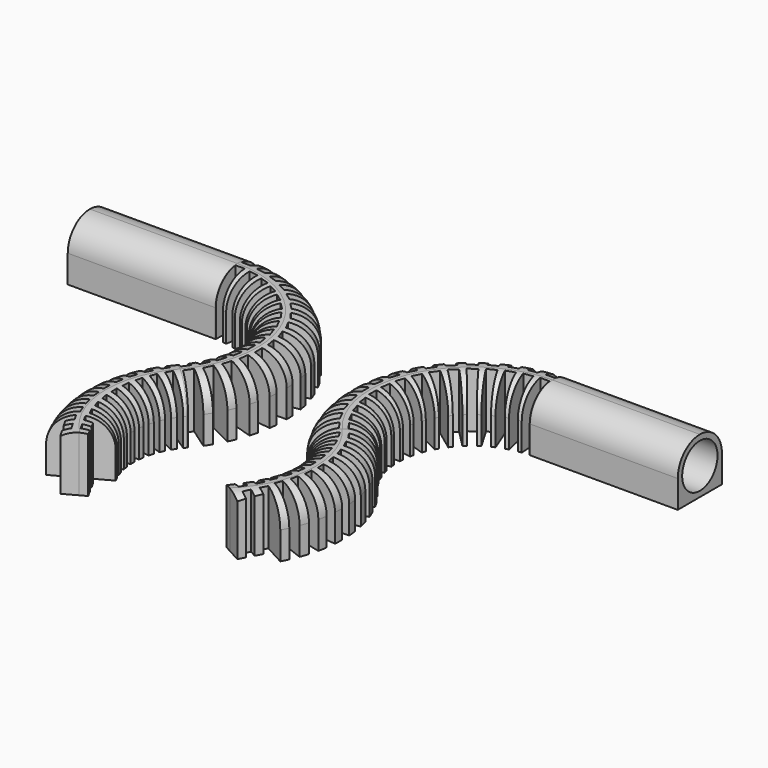
from build123d import *

# Parameters (mm, degrees)
F1_DEPTH = 15
F2_R     = 7.49999
F4_DEPTH = 15.0010001
F6_DEPTH = 25
F8_R     = 6
F9_DEPTH = 18


# Not quite as in the source:
# - a fillet or chamfer is up to 0.001 mm smaller than in the source, because OpenCascade refuses the exact size


with BuildPart() as f1:
    # F0 (on Top) → F1 (new body)
    with BuildSketch(Plane.XY):
        with BuildLine():
            Line((-77.8706056387, 57.7877178192), (-77.8706056387, 42.7877178192))
            Line((-77.8706056387, 42.7877178192), (-37.8706056387, 42.7877178192))
            ThreePointArc((-37.8706056387, 42.7877178192), (-19.7095136662, 31.1417172644), (-22.7163445519, 9.7778796274))
            ThreePointArc((-22.7163445519, 9.7778796274), (-30.7004171335, -8.6672744837), (-26.8147589411, -28.3870814195))
            Line((-26.8147589411, -28.3870814195), (-21.1033173398, -25.2839110882))
            Line((-21.1033173398, -25.2839110882), (-20.1484983127, -27.041272925))
            Line((-20.1484983127, -27.041272925), (-21.9058601495, -27.9960919522))
            Line((-21.9058601495, -27.9960919522), (-20.9510411223, -29.7534537889))
            Line((-20.9510411223, -29.7534537889), (-19.1936792855, -28.7986347618))
            Line((-19.1936792855, -28.7986347618), (-18.2388602584, -30.5559965986))
            Line((-18.2388602584, -30.5559965986), (-19.9962220952, -31.5108156257))
            Line((-19.9962220952, -31.5108156257), (-19.0414030681, -33.2681774625))
            Line((-19.0414030681, -33.2681774625), (-17.2840412313, -32.3133584354))
            Line((-17.2840412313, -32.3133584354), (-15.5266793945, -31.3585394083))
            Line((-15.5266793945, -31.3585394083), (-13.7693175577, -30.4037203811))
            Line((-13.7693175577, -30.4037203811), (-14.7241365848, -28.6463585444))
            Line((-14.7241365848, -28.6463585444), (-16.4814984216, -29.6011775715))
            Line((-16.4814984216, -29.6011775715), (-17.4363174487, -27.8438157347))
            Line((-17.4363174487, -27.8438157347), (-15.6789556119, -26.8889967076))
            Line((-15.6789556119, -26.8889967076), (-16.6337746391, -25.1316348708))
            Line((-16.6337746391, -25.1316348708), (-18.3911364759, -26.0864538979))
            Line((-18.3911364759, -26.0864538979), (-19.345955503, -24.3290920611))
            Line((-19.345955503, -24.3290920611), (-13.6345139017, -21.2259217298))
            ThreePointArc((-13.6345139017, -21.2259217298), (-15.7848603657, -10.2567502329), (-11.3412370802, 0))
            ThreePointArc((-11.3412370802, 0), (-6.0774156176, 37.3999840208), (-37.8706056387, 57.7877178192))
            Line((-37.8706056387, 57.7877178192), (-77.8706056387, 57.7877178192))
        make_face()
    extrude(amount=F1_DEPTH)

    # F2 (radius 7.5 in the source; OpenCascade refuses exactly that, so slightly less here)
    f2_edges = [f1.edges().sort_by_distance(p)[0] for p in [
        (-57.870606, 42.787718, 15),
        (-57.870606, 57.787718, 15),
    ]]
    fillet(f2_edges, radius=F2_R)

    # F3 (on Top) → F4 (cut, through all)
    with BuildSketch(Plane.XY):
        Polygon((-37.5368123768, 59.7073026001), (-37.5368123768, 51.4973428231), (-35.0368123768, 51.4973428231), (-34.0368123768, 59.7073026001), align=None)
        Polygon((-37.6518149255, 49.4973428231), (-37.6518149255, 33.8171138912), (-36.1518149255, 33.8171138912), (-35.1518149255, 49.4973428231), align=None)
        Polygon((-33.1543082816, 51.1186245676), (-30.6846017961, 50.7306169963), (-28.4225085803, 58.6858903306), (-31.88009766, 59.2291009305), align=None)
        Polygon((-36.0119423734, 33.6704828881), (-34.5301184821, 33.4376783452), (-31.1086168694, 48.7727005517), (-33.5783233549, 49.1607081231), align=None)
        Polygon((-28.8836869872, 50.0643174867), (-26.5041268876, 49.2977056344), (-23.0347618588, 56.8054979755), (-26.3661459983, 57.8787545688), align=None)
        Polygon((-34.4146983982, 33.2711154858), (-32.9869623384, 32.8111483744), (-27.22687856, 47.4293224814), (-29.6064386596, 48.1959343338), align=None)
        Polygon((-24.8284461961, 48.3599725139), (-22.5967006729, 47.2333350744), (-18.0041432391, 54.1116964895), (-21.1285869714, 55.6889889048), align=None)
        Polygon((-32.8987919068, 32.6286902782), (-31.5597445929, 31.9527078145), (-23.6006731938, 45.4997651267), (-25.8324187169, 46.6264025662), align=None)
        Polygon((-21.0868639046, 46.0468941285), (-19.0570188903, 44.5875349479), (-13.4525688155, 50.669769644), (-16.2943518355, 52.7128724969), align=None)
        Polygon((-31.5009606073, 31.758776319), (-30.2830535988, 30.8831608106), (-20.3178811748, 43.0307909466), (-22.3477261891, 44.4901501272), align=None)
        Polygon((-17.7496166548, 43.1811393493), (-15.9708650608, 41.4244257224), (-9.4903451366, 46.5631318877), (-11.9805973682, 49.0225309653), align=None)
        Polygon((-30.255080678, 30.6824558092), (-29.1878297216, 29.6284276331), (-17.458060349, 40.082235065), (-19.236811943, 41.8389486919), align=None)
        Polygon((-14.8975820049, 39.8321592036), (-13.413031541, 37.8206647541), (-6.2134959468, 41.8913068127), (-8.2918665963, 44.7073990419), align=None)
        Polygon((-29.1913457841, 29.4258131736), (-28.3006155058, 28.2189165039), (-15.0905179353, 36.7255551783), (-16.5750683992, 38.7370496278), align=None)
        Polygon((-12.5998784774, 36.081115594), (-11.4455069443, 33.8635885111), (-3.7014350689, 36.7675152197), (-5.3175552152, 39.8720531358), align=None)
        Polygon((-28.3355353405, 28.0193029096), (-27.6429124206, 26.6887866598), (-13.272630878, 33.0420997912), (-14.4270024111, 35.2596268741), align=None)
        Polygon((-10.9121904843, 32.0189143559), (-10.1159738587, 29.6490959905), (-2.0150418248, 31.3159312324), (-3.1297451007, 34.633676944), align=None)
        Polygon((-27.7083897519, 26.4970115285), (-27.2306597765, 25.0751205092), (-12.0484553275, 29.1211367508), (-12.8446719531, 31.4909551162), align=None)
        Polygon((-9.8754188262, 27.7440021709), (-9.4566532679, 25.2793246246), (-1.1951856373, 25.6686729618), (-1.7814574188, 29.1192215266), align=None)
        Polygon((-27.3251077736, 24.8958314751), (-27.0738484386, 23.4170249474), (-11.4476589476, 25.0576898578), (-11.8664245059, 27.5223674041), align=None)
        Polygon((-9.5146894689, 23.3599807303), (-9.4835236824, 20.8601749991), (-1.2617355664, 19.962600648), (-1.3053676675, 23.4623286717), align=None)
        Polygon((-27.1949781721, 23.2545670464), (-27.1762787002, 21.7546836077), (-11.4848019253, 20.950235982), (-11.5159677118, 23.4500417132), align=None)
        Polygon((-9.8387446204, 18.9730959677), (-10.1959339026, 16.4987443725), (-2.2130787872, 14.3359998785), (-1.7130137921, 17.8000921117), align=None)
        Polygon((-27.3211546137, 21.6129939766), (-27.5354681831, 20.1283830194), (-12.1589841076, 16.8983184943), (-11.8017948254, 19.3726700895), align=None)
        Polygon((-10.8397308651, 14.689663209), (-11.5766188011, 12.3007311945), (-4.026159676, 8.9252302628), (-2.9945165656, 12.269735083), align=None)
        Polygon((-27.7005792363, 20.0108954796), (-28.1427119979, 18.5775362709), (-13.4538668164, 13.0001348515), (-12.7169788804, 15.389066866), align=None)
        Polygon((-12.49338949, 10.6134906399), (-13.5921177395, 8.3678735234), (-6.6570385591, 3.8614207831), (-5.1188190097, 7.0052847461), align=None)
        Polygon((-28.3240567554, 18.4870981108), (-28.9832937051, 17.1397278409), (-15.3380688131, 9.3501567998), (-14.2393405636, 11.5957739162), align=None)
        Polygon((-14.7596443899, 6.8433635347), (-16.1935854808, 4.795483424), (-10.0419565823, -0.7327080918), (-8.0344390551, 2.1343240632), align=None)
        Polygon((-29.176477311, 17.0785308122), (-30.0368419655, 15.8498027458), (-17.7659268173, 6.0368408695), (-16.3319857265, 8.0847209802), align=None)
    extrude(amount=F4_DEPTH, mode=Mode.SUBTRACT)

    # F5 (on Top) → F6 (cut)
    with BuildSketch(Plane.XY):
        Polygon((-18.5813105237, 1.6833273234), (4.6174088509, -11.4270340175), (-17.6654999564, 3.3038495804), align=None)
        Polygon((-20.1421339034, -1.5767955582), (4.6174088509, -11.4270340175), (-19.4540558073, 0.1527563821), align=None)
        Polygon((-21.2474016708, -5.0181548809), (4.6174088509, -11.4270340175), (-20.7997161276, -3.2113956178), align=None)
        Polygon((-21.8767777904, -8.5774324096), (4.6174088509, -11.4270340175), (-21.6777218531, -6.7267087364), align=None)
        Polygon((-22.0186822495, -12.1891403089), (4.6174088509, -11.4270340175), (-22.0719183867, -10.3285040483), align=None)
        Polygon((-21.6705041205, -15.7868260673), (4.6174088509, -11.4270340175), (-21.9750528302, -13.9505114254), align=None)
        Polygon((-20.8386496, -19.3042951692), (4.6174088509, -11.4270340175), (-21.3889074317, -17.526088854), align=None)
        Polygon((-19.5384241402, -22.6768290207), (4.6174088509, -11.4270340175), (-20.3242667937, -20.9894485939), align=None)
        Polygon((-19.2797191247, 4.3709847051), (-26.4916419983, 9.1386744753), (-27.7598882718, 6.8704442901), (-20.3832731848, 2.7016758464), align=None)
        Polygon((-21.1978415938, 0.991619916), (-28.9886353394, 4.7394499672), (-29.9382517196, 2.3204531682), (-22.0653336642, -0.8116773798), align=None)
        Polygon((-22.6409842806, -2.616238087), (-30.8673045784, 0.0427751958), (-31.48081889, -2.4824806274), (-23.256453207, -4.5203446045), align=None)
        Polygon((-23.582594524, -6.3862076272), (-32.0930837168, -4.8649348121), (-32.3592077916, -7.4499869895), (-23.9347161747, -8.3560893426), align=None)
        Polygon((-24.0053474551, -10.2489243063), (-32.6434194075, -9.8933821515), (-32.557256777, -12.4906678086), (-24.0876430757, -12.2483369852), align=None)
        Polygon((-23.9014647609, -14.1333172538), (-32.5081859176, -14.9500474481), (-32.0713219048, -17.5117786239), (-23.7124201785, -16.1254733158), align=None)
        Polygon((-23.2728577994, -17.9679167729), (-31.6898714343, -19.9418921396), (-30.9103439845, -22.4209350473), (-22.8159512816, -19.9161621537), align=None)
        Polygon((-22.1310924313, -21.6821693261), (-30.2035322839, -24.7770703109), (-29.0956840734, -27.1278125608), (-21.4147306896, -23.5506578823), align=None)
    extrude(amount=F6_DEPTH, mode=Mode.SUBTRACT)

    # F8 (on face) → F9 (cut)
    with BuildSketch(Plane(origin=(-77.8706056387, 0, 0), x_dir=(0, -1, 0), z_dir=(-1, 0, 0))):
        with Locations((-50.2877178192, 7.5)):
            Circle(F8_R)
    extrude(amount=-F9_DEPTH, mode=Mode.SUBTRACT)


with BuildPart() as f10_1:
    # F10: instance of F1
    add(f1.part.mirror(Plane.YZ.offset(5)))


solid = Compound([f1.part, f10_1.part])
